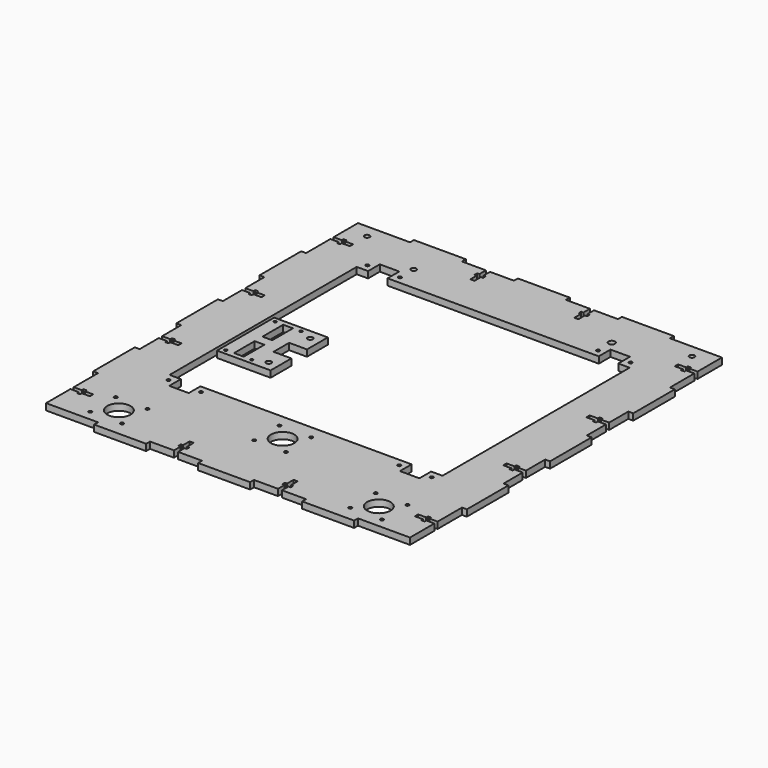
from build123d import *

# Parameters (mm, degrees)
F0_R     = 1.5875
F0_R_2   = 11.43
F0_W     = 41.275
F0_H     = 41.275
F0_R_3   = 3.175
F0_W_2   = 50.8
F0_H_2   = 4.7625
F0_W_3   = 4.7625
F0_H_3   = 50.8
F1_DEPTH = 6.35
F0_R_4   = 1.8415
F0_W_4   = 9.525
F0_H_4   = 25.273
F0_W_5   = 17.4625
F0_H_5   = 25.4
F2_D     = 2.7051
F3_D     = 5.1054
F4_D     = 5.1054


# Not quite as in the source:
# - a feature names something its author has since deleted; it is built from what else it names


with BuildPart() as f1:
    # F0 (on Top) → F1 (new body)
    with BuildSketch(Plane.XY):
        with BuildLine():
            ThreePointArc((155.575, 184.15), (158.75, 187.325), (161.925, 184.15))
            Line((161.925, 184.15), (177.8, 184.15))
            Line((177.8, 184.15), (177.8, 196.85))
            Line((177.8, 196.85), (127, 196.85))
            Line((127, 196.85), (76.2, 196.85))
            Line((76.2, 196.85), (52.7939, 196.85))
            Line((52.7939, 196.85), (52.7939, 188.8998))
            Line((52.7939, 188.8998), (54.9275, 188.8998))
            Line((54.9275, 188.8998), (54.9275, 185.7248))
            Line((54.9275, 185.7248), (52.7939, 185.7248))
            Line((52.7939, 185.7248), (52.7939, 184.15))
            Line((52.7939, 184.15), (155.575, 184.15))
        make_face()
        with BuildLine():
            ThreePointArc((155.575, 184.15), (158.75, 180.975), (161.925, 184.15))
            Line((161.925, 184.15), (155.575, 184.15))
        make_face()
        with BuildLine():
            Line((155.575, 184.15), (161.925, 184.15))
            ThreePointArc((161.925, 184.15), (158.75, 187.325), (155.575, 184.15))
        make_face()
        with BuildLine():
            Line((177.8, 184.15), (161.925, 184.15))
            ThreePointArc((161.925, 184.15), (158.75, 180.975), (155.575, 184.15))
            Line((155.575, 184.15), (52.7939, 184.15))
            Line((52.7939, 184.15), (52.7939, 177.8))
            Line((52.7939, 177.8), (48.8061, 177.8))
            Line((48.8061, 177.8), (48.8061, 184.15))
            Line((48.8061, 184.15), (-48.8061, 184.15))
            Line((-48.8061, 184.15), (-48.8061, 177.8))
            Line((-48.8061, 177.8), (-52.7939, 177.8))
            Line((-52.7939, 177.8), (-52.7939, 184.15))
            Line((-52.7939, 184.15), (-155.575, 184.15))
            ThreePointArc((-155.575, 184.15), (-158.75, 180.975), (-161.925, 184.15))
            Line((-161.925, 184.15), (-177.8, 184.15))
            Line((-177.8, 184.15), (-177.8, 167.0939))
            Line((-177.8, 167.0939), (-169.8498, 167.0939))
            Line((-169.8498, 167.0939), (-169.8498, 169.2275))
            Line((-169.8498, 169.2275), (-166.6748, 169.2275))
            Line((-166.6748, 169.2275), (-166.6748, 167.0939))
            Line((-166.6748, 167.0939), (-158.75, 167.0939))
            Line((-158.75, 167.0939), (-158.75, 163.1061))
            Line((-158.75, 163.1061), (-166.6748, 163.1061))
            Line((-166.6748, 163.1061), (-166.6748, 160.9725))
            Line((-166.6748, 160.9725), (-169.8498, 160.9725))
            Line((-169.8498, 160.9725), (-169.8498, 163.1061))
            Line((-169.8498, 163.1061), (-177.8, 163.1061))
            Line((-177.8, 163.1061), (-177.8, 133.35))
            Line((-177.8, 133.35), (-177.8, 82.55))
            Line((-177.8, 82.55), (-177.8, 59.1439))
            Line((-177.8, 59.1439), (-169.8498, 59.1439))
            Line((-169.8498, 59.1439), (-169.8498, 61.2775))
            Line((-169.8498, 61.2775), (-166.6748, 61.2775))
            Line((-166.6748, 61.2775), (-166.6748, 59.1439))
            Line((-166.6748, 59.1439), (-158.75, 59.1439))
            Line((-158.75, 59.1439), (-158.75, 55.1561))
            Line((-158.75, 55.1561), (-166.6748, 55.1561))
            Line((-166.6748, 55.1561), (-166.6748, 53.0225))
            Line((-166.6748, 53.0225), (-169.8498, 53.0225))
            Line((-169.8498, 53.0225), (-169.8498, 55.1561))
            Line((-169.8498, 55.1561), (-177.8, 55.1561))
            Line((-177.8, 55.1561), (-177.8, 31.75))
            Line((-177.8, 31.75), (-177.8, -19.05))
            Line((-177.8, -19.05), (-177.8, -42.4561))
            Line((-177.8, -42.4561), (-169.8498, -42.4561))
            Line((-169.8498, -42.4561), (-169.8498, -40.3225))
            Line((-169.8498, -40.3225), (-166.6748, -40.3225))
            Line((-166.6748, -40.3225), (-166.6748, -42.4561))
            Line((-166.6748, -42.4561), (-158.75, -42.4561))
            Line((-158.75, -42.4561), (-158.75, -46.4439))
            Line((-158.75, -46.4439), (-166.6748, -46.4439))
            Line((-166.6748, -46.4439), (-166.6748, -48.5775))
            Line((-166.6748, -48.5775), (-169.8498, -48.5775))
            Line((-169.8498, -48.5775), (-169.8498, -46.4439))
            Line((-169.8498, -46.4439), (-177.8, -46.4439))
            Line((-177.8, -46.4439), (-177.8, -69.85))
            Line((-177.8, -69.85), (-177.8, -120.65))
            Line((-177.8, -120.65), (-177.8, -150.4061))
            Line((-177.8, -150.4061), (-169.8498, -150.4061))
            Line((-169.8498, -150.4061), (-169.8498, -148.2725))
            Line((-169.8498, -148.2725), (-166.6748, -148.2725))
            Line((-166.6748, -148.2725), (-166.6748, -150.4061))
            Line((-166.6748, -150.4061), (-158.75, -150.4061))
            Line((-158.75, -150.4061), (-158.75, -154.3939))
            Line((-158.75, -154.3939), (-166.6748, -154.3939))
            Line((-166.6748, -154.3939), (-166.6748, -156.5275))
            Line((-166.6748, -156.5275), (-169.8498, -156.5275))
            Line((-169.8498, -156.5275), (-169.8498, -154.3939))
            Line((-169.8498, -154.3939), (-177.8, -154.3939))
            Line((-177.8, -154.3939), (-177.8, -184.15))
            Line((-177.8, -184.15), (-127, -184.15))
            Line((-127, -184.15), (-76.2, -184.15))
            Line((-76.2, -184.15), (-52.7939, -184.15))
            Line((-52.7939, -184.15), (-52.7939, -176.1998))
            Line((-52.7939, -176.1998), (-54.9275, -176.1998))
            Line((-54.9275, -176.1998), (-54.9275, -173.0248))
            Line((-54.9275, -173.0248), (-52.7939, -173.0248))
            Line((-52.7939, -173.0248), (-52.7939, -165.1))
            Line((-52.7939, -165.1), (-48.8061, -165.1))
            Line((-48.8061, -165.1), (-48.8061, -173.0248))
            Line((-48.8061, -173.0248), (-46.6725, -173.0248))
            Line((-46.6725, -173.0248), (-46.6725, -176.1998))
            Line((-46.6725, -176.1998), (-48.8061, -176.1998))
            Line((-48.8061, -176.1998), (-48.8061, -184.15))
            Line((-48.8061, -184.15), (-25.4, -184.15))
            Line((-25.4, -184.15), (25.4, -184.15))
            Line((25.4, -184.15), (48.8061, -184.15))
            Line((48.8061, -184.15), (48.8061, -176.1998))
            Line((48.8061, -176.1998), (46.6725, -176.1998))
            Line((46.6725, -176.1998), (46.6725, -173.0248))
            Line((46.6725, -173.0248), (48.8061, -173.0248))
            Line((48.8061, -173.0248), (48.8061, -165.1))
            Line((48.8061, -165.1), (52.7939, -165.1))
            Line((52.7939, -165.1), (52.7939, -173.0248))
            Line((52.7939, -173.0248), (54.9275, -173.0248))
            Line((54.9275, -173.0248), (54.9275, -176.1998))
            Line((54.9275, -176.1998), (52.7939, -176.1998))
            Line((52.7939, -176.1998), (52.7939, -184.15))
            Line((52.7939, -184.15), (76.2, -184.15))
            Line((76.2, -184.15), (127, -184.15))
            Line((127, -184.15), (177.8, -184.15))
            Line((177.8, -184.15), (177.8, -154.3939))
            Line((177.8, -154.3939), (169.8498, -154.3939))
            Line((169.8498, -154.3939), (169.8498, -156.5275))
            Line((169.8498, -156.5275), (166.6748, -156.5275))
            Line((166.6748, -156.5275), (166.6748, -154.3939))
            Line((166.6748, -154.3939), (158.75, -154.3939))
            Line((158.75, -154.3939), (158.75, -150.4061))
            Line((158.75, -150.4061), (166.6748, -150.4061))
            Line((166.6748, -150.4061), (166.6748, -148.2725))
            Line((166.6748, -148.2725), (169.8498, -148.2725))
            Line((169.8498, -148.2725), (169.8498, -150.4061))
            Line((169.8498, -150.4061), (177.8, -150.4061))
            Line((177.8, -150.4061), (177.8, -120.65))
            Line((177.8, -120.65), (177.8, -69.85))
            Line((177.8, -69.85), (177.8, -46.4439))
            Line((177.8, -46.4439), (169.8498, -46.4439))
            Line((169.8498, -46.4439), (169.8498, -48.5775))
            Line((169.8498, -48.5775), (166.6748, -48.5775))
            Line((166.6748, -48.5775), (166.6748, -46.4439))
            Line((166.6748, -46.4439), (158.75, -46.4439))
            Line((158.75, -46.4439), (158.75, -42.4561))
            Line((158.75, -42.4561), (166.6748, -42.4561))
            Line((166.6748, -42.4561), (166.6748, -40.3225))
            Line((166.6748, -40.3225), (169.8498, -40.3225))
            Line((169.8498, -40.3225), (169.8498, -42.4561))
            Line((169.8498, -42.4561), (177.8, -42.4561))
            Line((177.8, -42.4561), (177.8, -19.05))
            Line((177.8, -19.05), (177.8, 31.75))
            Line((177.8, 31.75), (177.8, 55.1561))
            Line((177.8, 55.1561), (169.8498, 55.1561))
            Line((169.8498, 55.1561), (169.8498, 53.0225))
            Line((169.8498, 53.0225), (166.6748, 53.0225))
            Line((166.6748, 53.0225), (166.6748, 55.1561))
            Line((166.6748, 55.1561), (158.75, 55.1561))
            Line((158.75, 55.1561), (158.75, 59.1439))
            Line((158.75, 59.1439), (166.6748, 59.1439))
            Line((166.6748, 59.1439), (166.6748, 61.2775))
            Line((166.6748, 61.2775), (169.8498, 61.2775))
            Line((169.8498, 61.2775), (169.8498, 59.1439))
            Line((169.8498, 59.1439), (177.8, 59.1439))
            Line((177.8, 59.1439), (177.8, 82.55))
            Line((177.8, 82.55), (177.8, 133.35))
            Line((177.8, 133.35), (177.8, 163.1061))
            Line((177.8, 163.1061), (169.8498, 163.1061))
            Line((169.8498, 163.1061), (169.8498, 160.9725))
            Line((169.8498, 160.9725), (166.6748, 160.9725))
            Line((166.6748, 160.9725), (166.6748, 163.1061))
            Line((166.6748, 163.1061), (158.75, 163.1061))
            Line((158.75, 163.1061), (158.75, 167.0939))
            Line((158.75, 167.0939), (166.6748, 167.0939))
            Line((166.6748, 167.0939), (166.6748, 169.2275))
            Line((166.6748, 169.2275), (169.8498, 169.2275))
            Line((169.8498, 169.2275), (169.8498, 167.0939))
            Line((169.8498, 167.0939), (177.8, 167.0939))
            Line((177.8, 167.0939), (177.8, 184.15))
        make_face()
        with Locations((-142.494, -174.244)):
            Circle(F0_R, mode=Mode.SUBTRACT)
        with Locations((-142.494, -143.256)):
            Circle(F0_R, mode=Mode.SUBTRACT)
        with Locations((-111.506, -174.244)):
            Circle(F0_R, mode=Mode.SUBTRACT)
        with Locations((-127, -158.75)):
            Circle(F0_R_2, mode=Mode.SUBTRACT)
        with Locations((-111.506, -143.256)):
            Circle(F0_R, mode=Mode.SUBTRACT)
        with Locations((-128.5875, -96.0501)):
            Circle(F0_R, mode=Mode.SUBTRACT)
        with Locations((-96.8375, -96.0501)):
            Circle(F0_R, mode=Mode.SUBTRACT)
        with Locations((0, -117.475)):
            Rectangle(F0_W, F0_H, mode=Mode.SUBTRACT)
        with Locations((111.506, -174.244)):
            Circle(F0_R, mode=Mode.SUBTRACT)
        with Locations((111.506, -143.256)):
            Circle(F0_R, mode=Mode.SUBTRACT)
        with Locations((127, -158.75)):
            Circle(F0_R_2, mode=Mode.SUBTRACT)
        with Locations((142.494, -174.244)):
            Circle(F0_R, mode=Mode.SUBTRACT)
        with Locations((142.494, -143.256)):
            Circle(F0_R, mode=Mode.SUBTRACT)
        with Locations((96.8375, -96.0501)):
            Circle(F0_R, mode=Mode.SUBTRACT)
        with Locations((128.5875, -96.0501)):
            Circle(F0_R, mode=Mode.SUBTRACT)
        with Locations((-128.5875, 146.8501)):
            Circle(F0_R, mode=Mode.SUBTRACT)
        with Locations((-96.8375, 146.8501)):
            Circle(F0_R, mode=Mode.SUBTRACT)
        with Locations((-96.8375, 163.5493947904)):
            Circle(F0_R_3, mode=Mode.SUBTRACT)
        Polygon((-122.2375, -88.9), (-133.35, -88.9), (-133.35, 139.7), (-122.2375, 139.7), (-122.2375, 154.0002), (-103.1875, 154.0002), (-103.1875, 139.7), (103.1875, 139.7), (103.1875, 154.0002), (122.2375, 154.0002), (122.2375, 139.7), (133.35, 139.7), (133.35, -88.9), (122.2375, -88.9), (122.2375, -103.2002), (103.1875, -103.2002), (103.1875, -88.9), (-103.1875, -88.9), (-103.1875, -103.2002), (-122.2375, -103.2002), align=None, mode=Mode.SUBTRACT)
        with Locations((96.8375, 146.8501)):
            Circle(F0_R, mode=Mode.SUBTRACT)
        with Locations((128.5875, 146.8501)):
            Circle(F0_R, mode=Mode.SUBTRACT)
        with Locations((96.8375, 163.5493947904)):
            Circle(F0_R_3, mode=Mode.SUBTRACT)
        with Locations((101.6, 199.23125)):
            Rectangle(F0_W_2, F0_H_2)
        Polygon((-48.8061, 184.15), (48.8061, 184.15), (48.8061, 185.7248), (46.6725, 185.7248), (46.6725, 188.8998), (48.8061, 188.8998), (48.8061, 196.85), (25.4, 196.85), (-25.4, 196.85), (-48.8061, 196.85), (-48.8061, 188.8998), (-46.6725, 188.8998), (-46.6725, 185.7248), (-48.8061, 185.7248), align=None)
        with Locations((180.18125, 107.95)):
            Rectangle(F0_W_3, F0_H_3)
        with BuildLine():
            Line((-155.575, 184.15), (-52.7939, 184.15))
            Line((-52.7939, 184.15), (-52.7939, 185.7248))
            Line((-52.7939, 185.7248), (-54.9275, 185.7248))
            Line((-54.9275, 185.7248), (-54.9275, 188.8998))
            Line((-54.9275, 188.8998), (-52.7939, 188.8998))
            Line((-52.7939, 188.8998), (-52.7939, 196.85))
            Line((-52.7939, 196.85), (-76.2, 196.85))
            Line((-76.2, 196.85), (-127, 196.85))
            Line((-127, 196.85), (-177.8, 196.85))
            Line((-177.8, 196.85), (-177.8, 184.15))
            Line((-177.8, 184.15), (-161.925, 184.15))
            ThreePointArc((-161.925, 184.15), (-158.75, 187.325), (-155.575, 184.15))
        make_face()
        with BuildLine():
            ThreePointArc((-161.925, 184.15), (-158.75, 180.975), (-155.575, 184.15))
            Line((-155.575, 184.15), (-161.925, 184.15))
        make_face()
        with BuildLine():
            Line((-161.925, 184.15), (-155.575, 184.15))
            ThreePointArc((-155.575, 184.15), (-158.75, 187.325), (-161.925, 184.15))
        make_face()
        with Locations((0, 199.23125)):
            Rectangle(F0_W_2, F0_H_2)
        with Locations((180.18125, 6.35)):
            Rectangle(F0_W_3, F0_H_3)
        with Locations((-101.6, 199.23125)):
            Rectangle(F0_W_2, F0_H_2)
        with Locations((-180.18125, 107.95)):
            Rectangle(F0_W_3, F0_H_3)
        with Locations((180.18125, -95.25)):
            Rectangle(F0_W_3, F0_H_3)
        with Locations((-180.18125, 6.35)):
            Rectangle(F0_W_3, F0_H_3)
        with Locations((101.6, -186.53125)):
            Rectangle(F0_W_2, F0_H_2)
        with Locations((-180.18125, -95.25)):
            Rectangle(F0_W_3, F0_H_3)
        with Locations((0, -186.53125)):
            Rectangle(F0_W_2, F0_H_2)
        with Locations((-101.6, -186.53125)):
            Rectangle(F0_W_2, F0_H_2)
        with Locations((-96.8375, 163.5493947904)):
            Circle(F0_R_3)
        with Locations((0, -117.475)):
            Rectangle(F0_W, F0_H)
        with Locations((-15.494, -132.969)):
            Circle(F0_R, mode=Mode.SUBTRACT)
        with Locations((-15.494, -101.981)):
            Circle(F0_R, mode=Mode.SUBTRACT)
        with Locations((15.494, -132.969)):
            Circle(F0_R, mode=Mode.SUBTRACT)
        with Locations((0, -117.475)):
            Circle(F0_R_2, mode=Mode.SUBTRACT)
        with Locations((15.494, -101.981)):
            Circle(F0_R, mode=Mode.SUBTRACT)
    extrude(amount=F1_DEPTH)

    # F4 (through all)
    with Locations(Plane(origin=(0, 0, 0), x_dir=(1, 0, 0), z_dir=(0, 0, -1))):
        with Locations((-158.75, -184.15), (-96.8375, -163.5493947904), (158.75, -184.15)):
            Hole(F4_D / 2)


with BuildPart() as f1b:
    # F0 (on Top) → F1, piece 2 (new body)
    with BuildSketch(Plane.XY):
        Polygon((-100.0125, 34.925), (-130.175, 34.925), (-130.175, -34.925), (-100.0125, -34.925), (-95.25, -34.925), (-95.25, -9.525), (-95.25, 9.525), (-95.25, 34.925), align=None)
        with Locations((-125.4125, -30.1625)):
            Circle(F0_R_4, mode=Mode.SUBTRACT)
        with Locations((-100.0125, -30.1625)):
            Circle(F0_R_4, mode=Mode.SUBTRACT)
        with Locations((-112.7125, -17.399)):
            Rectangle(F0_W_4, F0_H_4, mode=Mode.SUBTRACT)
        with Locations((-125.4125, 30.1625)):
            Circle(F0_R_4, mode=Mode.SUBTRACT)
        with Locations((-112.7125, 17.399)):
            Rectangle(F0_W_4, F0_H_4, mode=Mode.SUBTRACT)
        with Locations((-100.0125, 30.1625)):
            Circle(F0_R_4, mode=Mode.SUBTRACT)
        with Locations((-86.51875, 22.225)):
            Rectangle(F0_W_5, F0_H_5)
        with Locations((-87.3125, 25.4)):
            Circle(F0_R_3, mode=Mode.SUBTRACT)
        with Locations((-86.51875, -22.225)):
            Rectangle(F0_W_5, F0_H_5)
        with Locations((-87.3125, -25.4)):
            Circle(F0_R_3, mode=Mode.SUBTRACT)
        with Locations((-87.3125, 25.4)):
            Circle(F0_R_3)
        with Locations((-87.3125, -25.4)):
            Circle(F0_R_3)
        with Locations((-125.4125, 30.1625)):
            Circle(F0_R_4)
        with Locations((-100.0125, 30.1625)):
            Circle(F0_R_4)
        with Locations((-125.4125, -30.1625)):
            Circle(F0_R_4)
        with Locations((-100.0125, -30.1625)):
            Circle(F0_R_4)
    extrude(amount=F1_DEPTH)

    # F2 (through all)
    with Locations(Plane(origin=(0, 0, 0), x_dir=(1, 0, 0), z_dir=(0, 0, -1))):
        with Locations((-125.4125, -30.1625), (-100.0125, -30.1625), (-100.0125, 30.1625), (-125.4125, 30.1625)):
            Hole(F2_D / 2)

    # F3 (through all)
    with Locations(Plane(origin=(0, 0, 0), x_dir=(1, 0, 0), z_dir=(0, 0, -1))):
        with Locations((-87.3125, -25.4), (-87.3125, 25.4)):
            Hole(F3_D / 2)


solid = Compound([f1.part, f1b.part])
